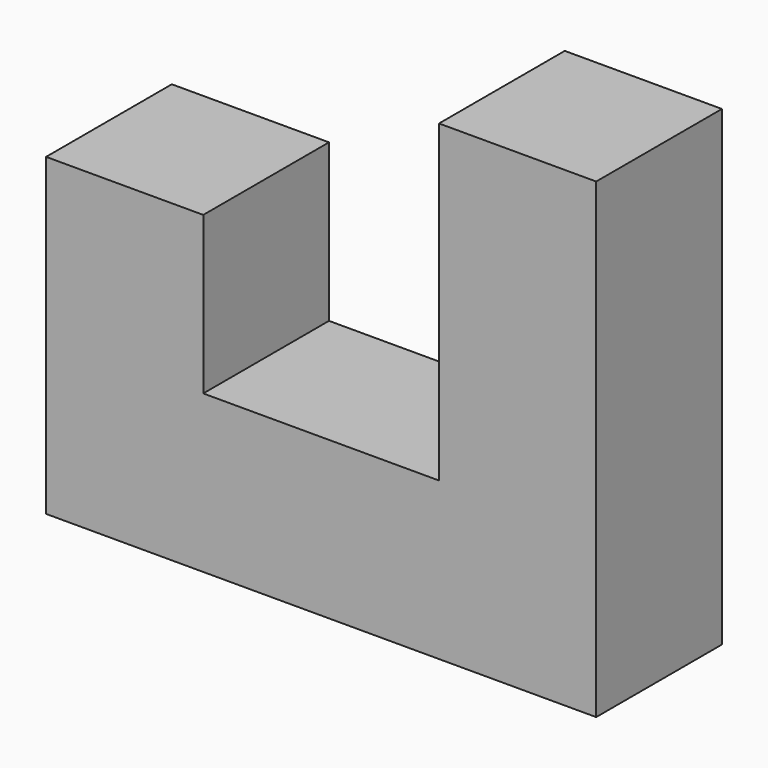
from build123d import *

# Parameters (mm, degrees)
F1_DEPTH = 25.4


# Not quite as in the source:
# - a feature names something its author has since deleted; it is built from what else it names


with BuildPart() as f1:
    # F0 (on Front) → F1 (new body)
    with BuildSketch(Plane.XZ):
        Polygon((-42.3630376343, 18.153519598), (-42.3630376343, -32.646480402), (46.5369623657, -32.646480402), (46.5369623657, 43.553519598), (21.1369623657, 43.553519598), (21.1369623657, -7.246480402), (-16.9630376343, -7.246480402), (-16.9630376343, 18.153519598), align=None)
    extrude(amount=F1_DEPTH)


solid = f1.part
